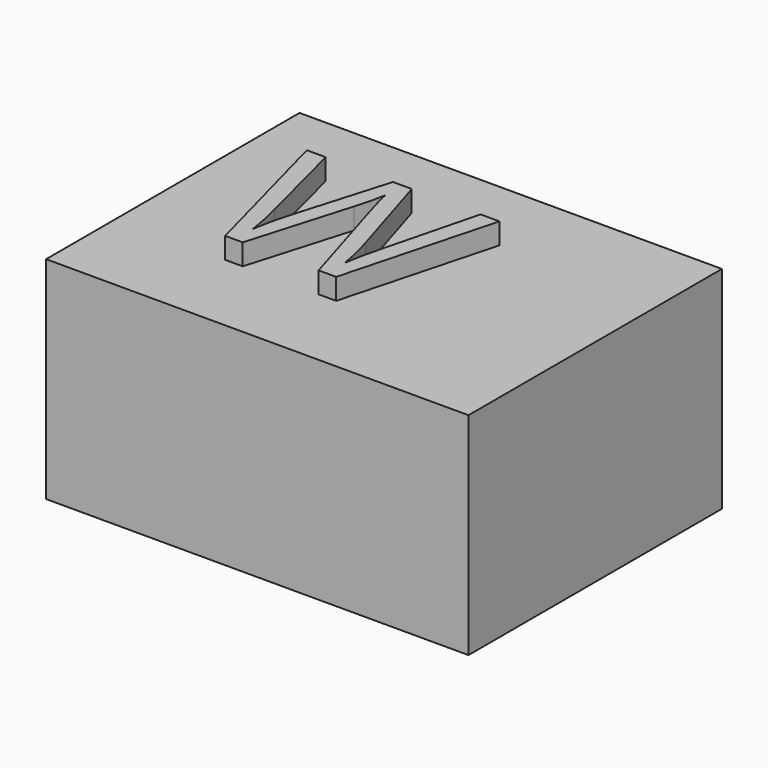
from build123d import *

# Parameters (mm, degrees)
F0_W         = 50.8
F0_H         = 38.1
F1_DEPTH     = 25.4
F2_TEXT_SIZE = 25.7643444153
F3_DEPTH     = 2.54


# Not quite as in the source:
# - Text() gives the source's letters only with a copy of the font that has no kerning and outlines rounded to 1/6400 em; it was checked with that copy


with BuildPart() as f1:
    # F0 (on Top) → F1 (new body)
    with BuildSketch(Plane.XY):
        with Locations((-25.4, 19.05)):
            Rectangle(F0_W, F0_H)
    extrude(amount=F1_DEPTH)

    # F2 (on face) → F3 (join)
    with BuildSketch(Plane.XY.offset(25.4)):
        with Locations((-42.8156554699, 10.3994263336)):
            Text('W', F2_TEXT_SIZE, font='Open Sans', text_align=(TextAlign.LEFT, TextAlign.BOTTOM))
    extrude(amount=F3_DEPTH)


solid = f1.part
